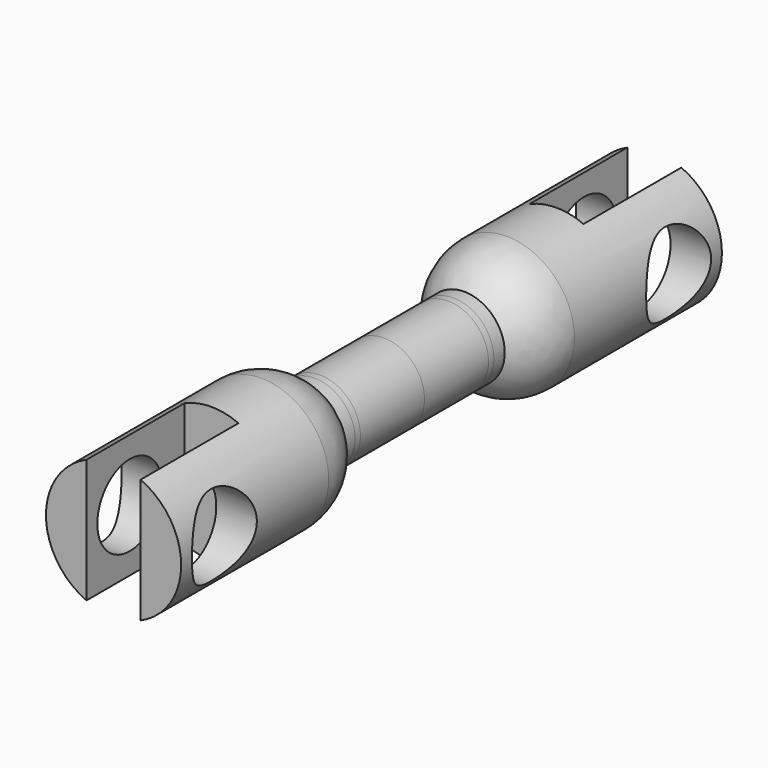
from build123d import *

# Parameters (mm, degrees)
F1_R          = 3
F2_DEPTH      = 15
F1_R_2        = 5
F3_DEPTH      = 10
F3_DEPTH_BACK = 8.58
F4_S5_R       = 3
F4_T6_DEPTH   = 13095
F6_DEPTH      = 9.05
F7_R          = 3
F8_DEPTH      = 25
F8_DEPTH_BACK = 25


# Not quite as in the source:
# - a fillet or chamfer that OpenCascade refuses, or shapes differently, is made with other operations: its cross-section is extruded or revolved along the edge and cut away or added


with BuildPart() as f2:
    # F1 (on Front) → F2 (new body)
    with BuildSketch(Plane.XZ):
        Circle(F1_R)
    extrude(amount=F2_DEPTH)

    # F1 (on Front) → F3 (join, two sides)
    with BuildSketch(Plane.XZ) as f3_sk:
        Circle(F1_R_2)
        Circle(F1_R, mode=Mode.SUBTRACT)
        Circle(F1_R)
    extrude(amount=-F3_DEPTH)
    extrude(f3_sk.sketch, amount=F3_DEPTH_BACK)

    # F4: fillet of radius 5 on 1 edges, made by hand


with BuildPart() as f4_tool2:
    # F4_s3 → F4_t4 (revolve)
    with BuildSketch(Plane.XY):
        with BuildLine():
            ThreePointArc((0, -8.5803999068), (3.5358753108, -7.1151924681), (5.0004, -3.5790343146))
            Line((5.0004, -3.5790343146), (5.5005365685, -3.5790343146))
            ThreePointArc((5.5005365685, -3.5790343146), (5.5001365685, -6.0795171573), (5.5001365685, -8.58))
            Line((5.5001365685, -8.58), (5, -9.0801365685))
            Line((5, -9.0801365685), (0, -9.0805364913))
            Line((0, -9.0805364913), (0, -8.5803999068))
        make_face()
    revolve(axis=Axis((0, -8.58, 0), (0, -1, 0)))

    # F4_s5 → F4_t6 (cut, symmetric)
    with BuildSketch(Plane.XZ.offset(7.3)):
        Circle(F4_S5_R)
    extrude(amount=F4_T6_DEPTH, both=True, mode=Mode.SUBTRACT)


with BuildPart() as f2_1:
    add(f2.part)

    # F4_t1: cut F4_tool2
    add(f4_tool2.part, mode=Mode.SUBTRACT)

    # F5 (on face) → F6 (cut)
    with BuildSketch(Plane(origin=(0, 10, 0), x_dir=(-1, 0, 0), z_dir=(0, 1, 0))):
        with BuildLine():
            Line((-2, 4.582575695), (-2, -4.582575695))
            ThreePointArc((-2, -4.582575695), (0, -5), (2, -4.582575695))
            Line((2, -4.582575695), (2, 4.582575695))
            ThreePointArc((2, 4.582575695), (0, 5), (-2, 4.582575695))
        make_face()
    extrude(amount=-F6_DEPTH, mode=Mode.SUBTRACT)

    # F7 (on face) → F8 (cut, two sides)
    with BuildSketch(Plane.YZ.offset(-2)) as f8_sk:
        with Locations((6, 0)):
            Circle(F7_R)
    extrude(amount=F8_DEPTH, mode=Mode.SUBTRACT)
    extrude(f8_sk.sketch, amount=-F8_DEPTH_BACK, mode=Mode.SUBTRACT)

    # F9: F2 across face


with BuildPart() as f2_2:
    add(f2_1.part)
    add(f2_1.part.mirror(Plane.XZ.offset(15)))


solid = f2_2.part
